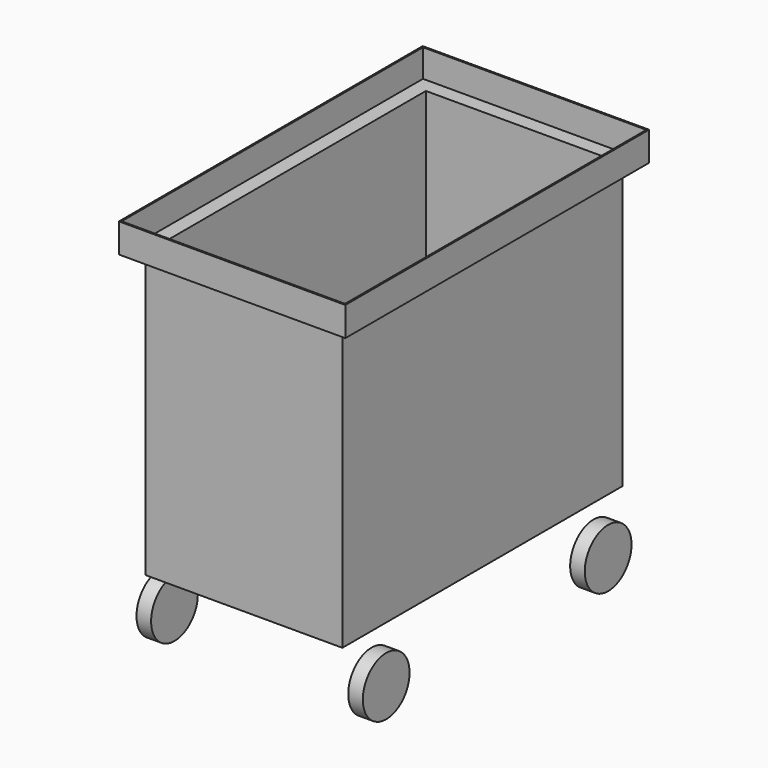
from build123d import *

# Parameters (mm, degrees)
F1_W     = 675
F1_H     = 1200
F2_DEPTH = 1070
F3_W     = 775
F3_H     = 1300
F3_W_2   = 675
F3_H_2   = 1200
F4_DEPTH = 100
F5_T     = -5
F6_R     = 100
F7_DEPTH = 50
F8_R     = 100
F9_DEPTH = 50


# Not quite as in the source:
# - a feature names something its author has since deleted; it is built from what else it names


with BuildPart() as f2:
    # F1 (on offset) → F2 (new body)
    with BuildSketch(Plane.XY.offset(250)):
        with Locations((387.5, 650)):
            Rectangle(F1_W, F1_H)
    extrude(amount=F2_DEPTH)

    # F3 (on face) → F4 (join)
    with BuildSketch(Plane.XY.offset(1320)):
        with Locations((387.5, 650)):
            Rectangle(F3_W, F3_H)
        with Locations((387.5, 650)):
            Rectangle(F3_W_2, F3_H_2, mode=Mode.SUBTRACT)
    extrude(amount=-F4_DEPTH)

    # F5
    f5_openings = [f2.faces().sort_by_distance(p)[0] for p in [
        (387.5, 650, 1320),
    ]]
    offset(amount=F5_T, openings=f5_openings, kind=Kind.INTERSECTION)


with BuildPart() as f7:
    # F6 (on Right) → F7 (new body, through all)
    with BuildSketch(Plane.YZ):
        with Locations((1125, 100)):
            Circle(F6_R)
    extrude(amount=F7_DEPTH)


with BuildPart() as f7b:
    # F6 (on Right) → F7, piece 2 (new body, through all)
    with BuildSketch(Plane.YZ):
        with Locations((175, 100)):
            Circle(F6_R)
    extrude(amount=F7_DEPTH)


with BuildPart() as f9:
    # F8 (on face) → F9 (new body, through all)
    with BuildSketch(Plane.YZ.offset(725)):
        with Locations((1125, 100)):
            Circle(F8_R)
    extrude(amount=F9_DEPTH)


with BuildPart() as f9b:
    # F8 (on face) → F9, piece 2 (new body, through all)
    with BuildSketch(Plane.YZ.offset(725)):
        with Locations((175, 100)):
            Circle(F8_R)
    extrude(amount=F9_DEPTH)


solid = Compound([f2.part, f7.part, f7b.part, f9.part, f9b.part])
